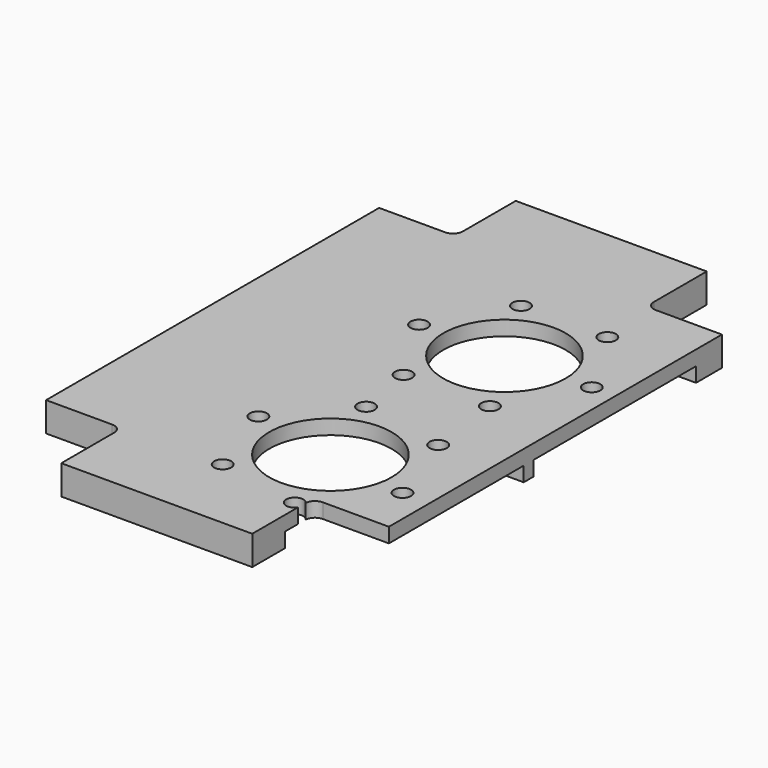
from build123d import *

# Parameters (mm, degrees)
F1_DEPTH     = 6
F3_DEPTH     = 3
F4_R         = 12.5
F5_DEPTH     = 25
F6_R         = 1.75
F7_DEPTH     = 25
F8_R         = 1.75
F9_DEPTH     = 25
F10_T1_DEPTH = 6
F10_T3_DEPTH = 3
F11_R        = 2


# Not quite as in the source:
# - a fillet or chamfer that OpenCascade refuses, or shapes differently, is made with other operations: its cross-section is extruded or revolved along the edge and cut away or added


with BuildPart() as f1:
    # F0 (on Top) → F1 (new body)
    with BuildSketch(Plane.XY):
        Polygon((15.5, -15.5), (0, -15.5), (0, -100.5), (15.5, -100.5), (15.5, -116), (54.5, -116), (54.5, -100.5), (70, -100.5), (70, -15.5), (54.5, -15.5), (54.5, 0), (15.5, 0), align=None)
    extrude(amount=F1_DEPTH)

    # F2 (on face) → F3 (cut)
    with BuildSketch(Plane(origin=(0, 0, 0), x_dir=(1, 0, 0), z_dir=(0, 0, -1))):
        with BuildLine():
            Line((46.0390912639, 107.6606247352), (48.3088987836, 107.6606247352))
            ThreePointArc((48.3088987836, 107.6606247352), (47.1739950237, 107.6916095092), (46.0390912639, 107.6606247352))
        make_face()
        with BuildLine():
            Line((46.863162711, 63.6384694919), (48.4956821186, 63.6384694919))
            ThreePointArc((48.4956821186, 63.6384694919), (47.6794224148, 63.6544920069), (46.863162711, 63.6384694919))
        make_face()
        with BuildLine():
            Line((54.5, 107.6606247352), (48.3088987836, 107.6606247352))
            Line((48.3088987836, 107.6606247352), (46.0390912639, 107.6606247352))
            ThreePointArc((46.0390912639, 107.6606247352), (26.3780814544, 86.4793246358), (46.863162711, 66.0939321564))
            Line((46.863162711, 66.0939321564), (70, 66.0939321564))
            Line((70, 66.0939321564), (70, 100.5))
            Line((70, 100.5), (54.5, 100.5))
            Line((54.5, 100.5), (54.5, 107.6606247352))
        make_face()
        with BuildLine():
            Line((70, 22.1093658845), (70, 63.6384694919))
            Line((70, 63.6384694919), (48.4956821186, 63.6384694919))
            Line((48.4956821186, 63.6384694919), (46.863162711, 63.6384694919))
            ThreePointArc((46.863162711, 63.6384694919), (26.8823229814, 43.2018465212), (46.1695409076, 22.1093658845))
            Line((46.1695409076, 22.1093658845), (70, 22.1093658845))
        make_face()
    extrude(amount=-F3_DEPTH, mode=Mode.SUBTRACT)

    # F4 (on face) → F5 (cut)
    with BuildSketch(Plane(origin=(0, 0, 3), x_dir=(1, 0, 0), z_dir=(0, 0, -1))):
        with Locations((47.51990363, 42.9035276175)):
            Circle(F4_R)
        with Locations((47.1739950237, 86.8916095092)):
            Circle(F4_R)
    extrude(amount=-F5_DEPTH, mode=Mode.SUBTRACT)

    # F6 (on face) → F7 (cut)
    with BuildSketch(Plane(origin=(0, 0, 3), x_dir=(1, 0, 0), z_dir=(0, 0, -1))):
        with Locations((39.0656358559, 58.0877674629)):
            Circle(F6_R)
        with Locations((30.1801256076, 43.0113717521)):
            Circle(F6_R)
        with Locations((38.7939121665, 27.7780962961)):
            Circle(F6_R)
        with Locations((56.2932089737, 27.6212165509)):
            Circle(F6_R)
        with Locations((65.178719222, 42.6976122617)):
            Circle(F6_R)
        with Locations((56.5649326631, 57.9308877176)):
            Circle(F6_R)
    extrude(amount=-F7_DEPTH, mode=Mode.SUBTRACT)

    # F8 (on face) → F9 (cut)
    with BuildSketch(Plane(origin=(0, 0, 3), x_dir=(1, 0, 0), z_dir=(0, 0, -1))):
        with Locations((35.8538748382, 100.2372035006)):
            Circle(F8_R)
        with Locations((29.9563115058, 83.7608948503)):
            Circle(F8_R)
        with Locations((41.2764316914, 70.4153008589)):
            Circle(F8_R)
        with Locations((58.4941152093, 73.5460155178)):
            Circle(F8_R)
        with Locations((64.3916785417, 90.0223241681)):
            Circle(F8_R)
        with Locations((53.0715583561, 103.3679181595)):
            Circle(F8_R)
    extrude(amount=-F9_DEPTH, mode=Mode.SUBTRACT)

    # F10: fillet of radius 2 on 2 edges, made by hand

    # F10_s2 → F10_t1 (join)
    with BuildSketch(Plane.XY):
        with BuildLine():
            ThreePointArc((13.5, -100.5), (14.9142135624, -101.0857864376), (15.5, -102.5))
            Line((15.5, -102.5), (15.5, -100.5))
            Line((15.5, -100.5), (13.5, -100.5))
        make_face()
    extrude(amount=F10_T1_DEPTH)

    # F10_s4 → F10_t3 (join)
    with BuildSketch(Plane.XY.offset(3)):
        with BuildLine():
            ThreePointArc((56.4948776909, -100.5), (55.1321777741, -101.0360843819), (54.5, -102.3569510631))
            Line((54.5, -102.3569510631), (54.5, -100.5))
            Line((54.5, -100.5), (56.4948776909, -100.5))
        make_face()
    extrude(amount=F10_T3_DEPTH)

    # F11
    f11_edges = [f1.edges().sort_by_distance(p)[0] for p in [
        (54.5, -15.5, 3),
        (15.5, -15.5, 3),
    ]]
    fillet(f11_edges, radius=F11_R)


solid = f1.part
